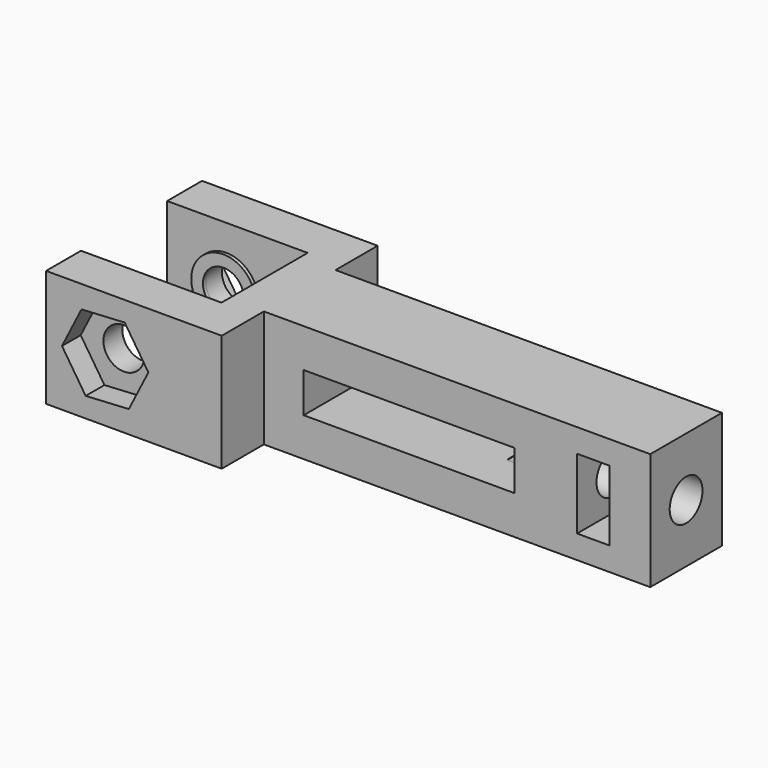
from build123d import *

# Parameters (mm, degrees)
F0_W      = 33
F0_H      = 3.825
F1_DEPTH  = 10
F2_R      = 1.75
F3_DEPTH  = 16.651
F4_W      = 18
F4_H      = 3.4
F4_W_2    = 2.75
F4_H_2    = 6
F5_DEPTH  = 12.151
F6_R      = 1.75
F7_DEPTH  = 15
F10_DEPTH = 2
F11_W     = 17.65
F11_H     = 60
F12_DEPTH = 8
F13_R     = 1.75
F14_DEPTH = 63.001
F15_R     = 2.75
F15_R_2   = 1.75
F16_DEPTH = 0.3
F17_R     = 1.75
F18_DEPTH = 2
F19_R     = 3.75
F20_DEPTH = 4


# Not quite as in the source:
# - a pattern or mirror of a feature is missing from the dataset's text; its kind, count and spacing are read off the source's solid


with BuildPart() as f1:
    # F0 (on Top) → F1 (new body)
    with BuildSketch(Plane.XY):
        Polygon((0, -3.825), (0, 0), (-3, 0), (-3, -4.6), (-15, -4.6), (-15, -8.325), (0, -8.325), align=None)
        Polygon((-3, 0), (0, 0), (0, 3.825), (0, 8.325), (-15, 8.325), (-15, 4.6), (-3, 4.6), align=None)
        with Locations((16.5, 1.9125)):
            Rectangle(F0_W, F0_H)
        with Locations((16.5, -1.9125)):
            Rectangle(F0_W, F0_H)
    extrude(amount=F1_DEPTH)

    # F2 (on face) → F3 (cut, through all)
    with BuildSketch(Plane.XZ.offset(8.325)):
        with Locations((-9.9527407438, 5)):
            Circle(F2_R)
    extrude(amount=-F3_DEPTH, mode=Mode.SUBTRACT)

    # F4 (on face) → F5 (cut, through all)
    with BuildSketch(Plane.XZ.offset(3.825)):
        with Locations((12.4002694301, 5)):
            Rectangle(F4_W, F4_H)
        with Locations((28.125, 5)):
            Rectangle(F4_W_2, F4_H_2)
    extrude(amount=-F5_DEPTH, mode=Mode.SUBTRACT)

    # F6 (on face) → F7 (cut)
    with BuildSketch(Plane.YZ.offset(33)):
        with Locations((0, 5)):
            Circle(F6_R)
    extrude(amount=-F7_DEPTH, mode=Mode.SUBTRACT)

    # F15 (on face) → F16 (join)
    with BuildSketch(Plane.XZ.offset(-4.6)):
        with Locations((-9.9527407438, 5)):
            Circle(F15_R)
        with Locations((-9.9527407438, 5)):
            Circle(F15_R_2, mode=Mode.SUBTRACT)
    f16 = extrude(amount=F16_DEPTH)

    # F16_copies: F16 across plane
    add(f16.mirror(Plane(origin=(0, 0, 0), x_dir=(0, 0, -1), z_dir=(0, -1, 0))))

    # F17 (on face) → F18 (cut)
    with BuildSketch(Plane.XZ.offset(8.325)):
        Polygon((-7.9284293953, 1.9088033227), (-6.2635302189, 5.2075067143), (-8.2878415673, 8.2987033916), (-11.9770520922, 8.0911966773), (-13.6419512686, 4.7924932857), (-11.6176399202, 1.7012966084), align=None)
        with Locations((-9.9527407438, 5)):
            Circle(F17_R, mode=Mode.SUBTRACT)
    f18 = extrude(amount=-F18_DEPTH, mode=Mode.SUBTRACT)

    # F18_copies: F18 across plane
    add(f18.mirror(Plane.ZX), mode=Mode.SUBTRACT)


with BuildPart() as f10:
    # F9 (on offset) → F10 (new body)
    with BuildSketch(Plane.YZ.offset(38)):
        Polygon((3.825, 0), (3.825, 10), (3.825, 19.8484882712), (-3.825, 19.8484882712), (-3.825, 10), (-3.825, 0), (-3.825, -10.1515117288), (3.825, -10.1515117288), align=None)
    extrude(amount=F10_DEPTH)

    # F11 (on face) → F12 (join)
    with BuildSketch(Plane.YZ.offset(40)):
        with Locations((0, 4.8484882712)):
            Rectangle(F11_W, F11_H)
    extrude(amount=F12_DEPTH)

    # F13 (on face) → F14 (cut, through all)
    with BuildSketch(Plane.YZ.offset(48)):
        with Locations((0, 5)):
            Circle(F13_R)
    extrude(amount=-F14_DEPTH, mode=Mode.SUBTRACT)

    # F19 (on face) → F20 (join)
    with BuildSketch(Plane(origin=(40, 0, 0), x_dir=(0, -1, 0), z_dir=(-1, 0, 0))):
        with Locations((0, 28)):
            Circle(F19_R)
        with Locations((0, -18)):
            Circle(F19_R)
    extrude(amount=F20_DEPTH)


solid = f1.part
